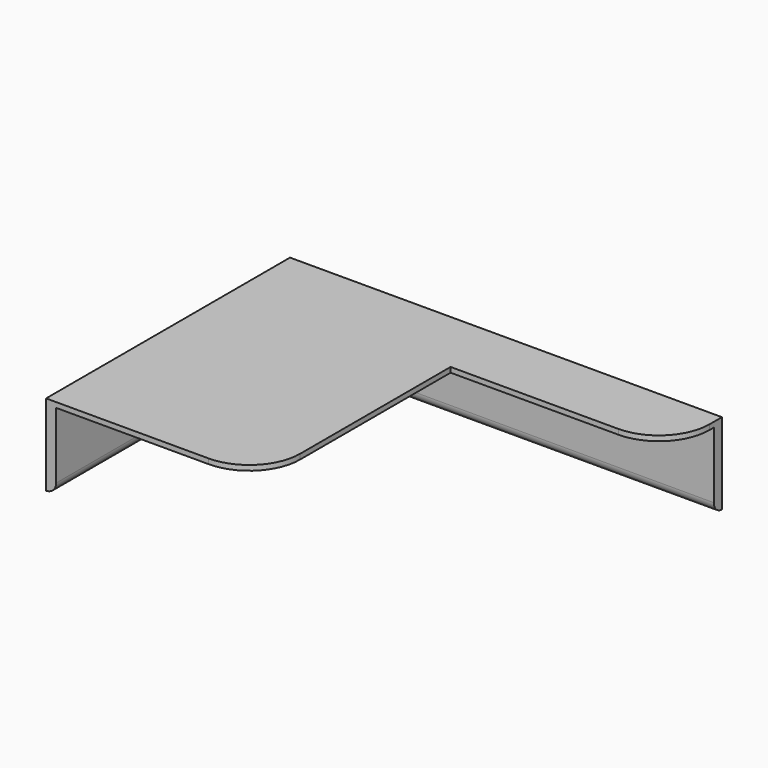
from build123d import *

# Parameters (mm, degrees)
F1_DEPTH = 1
F3_DEPTH = 15
F4_R     = 1.99999
F5_R     = 10


# Not quite as in the source:
# - a fillet or chamfer is up to 0.001 mm smaller than in the source, because OpenCascade refuses the exact size


with BuildPart() as f1:
    # F0 (on Top) → F1 (new body)
    with BuildSketch(Plane.XY):
        Polygon((-42, -47), (0, -47), (0, 0), (43, 0), (43, 13), (-42, 13), (-42, 0), align=None)
    extrude(amount=F1_DEPTH)

    # F2 (on face) → F3 (join)
    with BuildSketch(Plane(origin=(0, 0, 0), x_dir=(1, 0, 0), z_dir=(0, 0, -1))):
        Polygon((-42, 47), (-42, -13), (-40, -13), (43, -13), (43, -11), (-40, -11), (-40, 47), align=None)
    extrude(amount=F3_DEPTH)

    # F4 (radius 2 in the source; OpenCascade refuses exactly that, so slightly less here)
    f4_edges = [f1.edges().sort_by_distance(p)[0] for p in [
        (-40, -18, -15),
        (1.5, 11, -15),
    ]]
    fillet(f4_edges, radius=F4_R)

    # F5
    f5_edges = [f1.edges().sort_by_distance(p)[0] for p in [
        (0, -47, 0.5),
        (43, 0, 0.5),
    ]]
    fillet(f5_edges, radius=F5_R)


solid = f1.part
